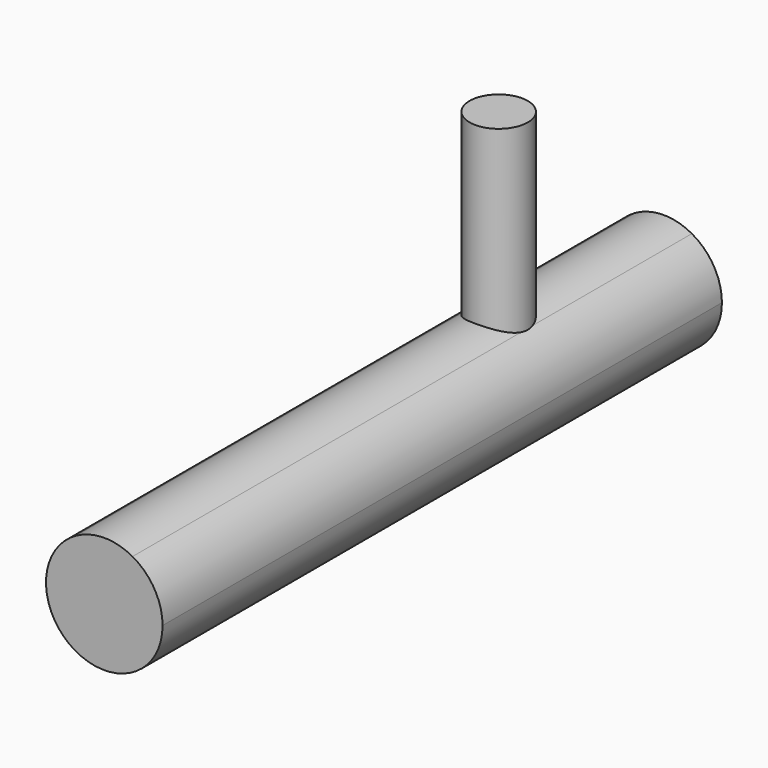
from build123d import *
from build123d import SkipClean  # not in build123d's __all__

# Parameters (mm, degrees)
F1_DEPTH = 76.2
F2_R     = 3.175
F3_DEPTH = 25.4


with BuildPart() as f1:
    # F0 (on Front) → F1 (new body)
    with BuildSketch(Plane.XZ):
        with BuildLine():
            ThreePointArc((-3.0741805311, 5.55625), (-3.2250157851, -5.4700798153), (6.35, 0))
            ThreePointArc((6.35, 0), (5.4700798153, 3.2250157851), (3.0741805311, 5.55625))
            ThreePointArc((3.0741805311, 5.55625), (0, 6.35), (-3.0741805311, 5.55625))
        make_face()
    extrude(amount=F1_DEPTH)

    # F2 (on Top) → F3 (join)
    with BuildSketch(Plane.XY):
        with Locations((0, -22.4732574466)):
            Circle(F2_R)
    with SkipClean():  # cleaning this boolean's faces spoils the solid; the shape is the same uncleaned
        extrude(amount=F3_DEPTH)


solid = f1.part
